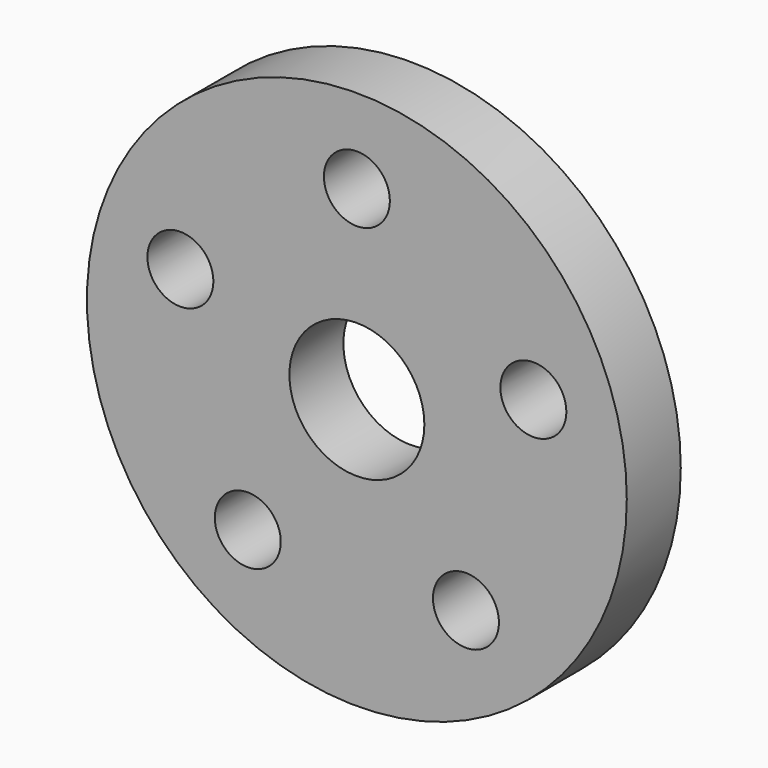
from build123d import *

# Parameters (mm, degrees)
F0_R            = 40
F1_DEPTH        = 10
F2_R            = 4.8873689042
F3_DEPTH        = 25
F3_COPIES_COUNT = 5
F4_R            = 10
F5_DEPTH        = 25


# Not quite as in the source:
# - a pattern or mirror of a feature is missing from the dataset's text; its kind, count and spacing are read off the source's solid


with BuildPart() as f1:
    # F0 (on Front) → F1 (new body)
    with BuildSketch(Plane.XZ):
        Circle(F0_R)
    extrude(amount=F1_DEPTH)

    # F2 (on face) → F3 (cut)
    with BuildSketch(Plane.XZ.offset(10)):
        with Locations((0, 27.5)):
            Circle(F2_R)
    f3 = extrude(amount=-F3_DEPTH, mode=Mode.SUBTRACT)

    # F3_copies: F3 ×5 about axis
    f3_copies_axis = Axis((0, 0, 0), (0, 1, 0))
    for i in range(1, F3_COPIES_COUNT):
        add(f3.rotate(f3_copies_axis, i * 360 / F3_COPIES_COUNT), mode=Mode.SUBTRACT)

    # F4 (on face) → F5 (cut)
    with BuildSketch(Plane.XZ.offset(10)):
        Circle(F4_R)
    extrude(amount=-F5_DEPTH, mode=Mode.SUBTRACT)


solid = f1.part
